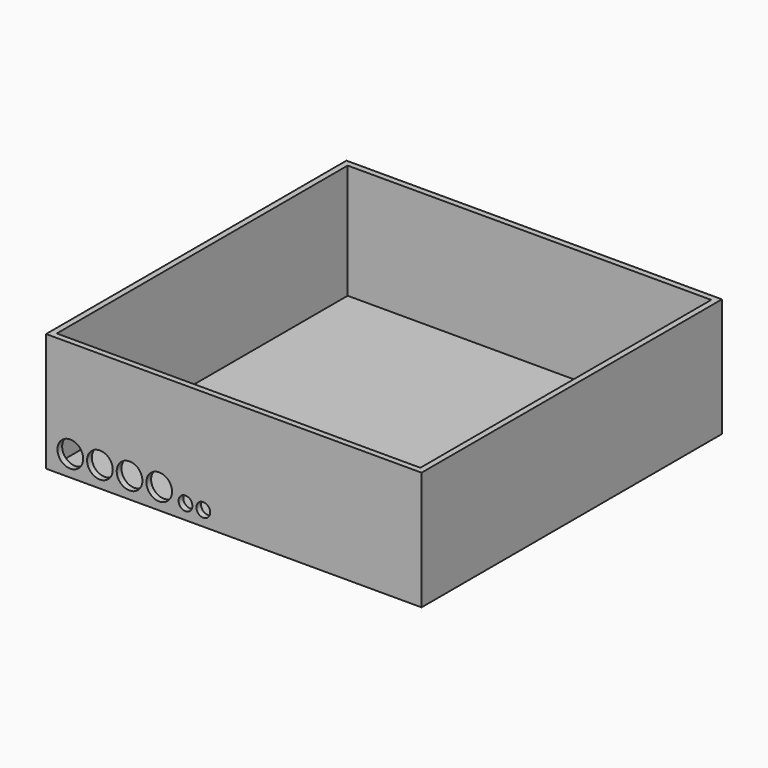
from build123d import *

# Parameters (mm, degrees)
F0_W     = 184
F0_H     = 184
F1_DEPTH = 2
F0_W_2   = 190
F0_H_2   = 190
F2_DEPTH = 60
F3_R     = 3.5
F3_R_2   = 6.5
F4_DEPTH = 4
F5_DEPTH = 3
F6_SIZE  = 2


# Not quite as in the source:
# - a feature names something its author has since deleted; it is built from what else it names


with BuildPart() as f1:
    # F0 (on Top) → F1 (new body)
    with BuildSketch(Plane.XY):
        with Locations((35.6310763971, 41.0211185324)):
            Rectangle(F0_W, F0_H)
    extrude(amount=F1_DEPTH)

    # F0 (on Top) → F2 (join)
    with BuildSketch(Plane.XY):
        with Locations((35.6310763971, 41.0211185324)):
            Rectangle(F0_W_2, F0_H_2)
        with Locations((35.6310763971, 41.0211185324)):
            Rectangle(F0_W, F0_H, mode=Mode.SUBTRACT)
    extrude(amount=F2_DEPTH)

    # F3 (on face) → F4 (cut)
    with BuildSketch(Plane.XZ.offset(53.9788814676)):
        with Locations((20.1768895756, 7.5)):
            Circle(F3_R)
        with Locations((11.1768895756, 7.5)):
            Circle(F3_R)
        with Locations((-32.1242534935, 10.5)):
            Circle(F3_R_2)
        with Locations((-47.1242534935, 10.5)):
            Circle(F3_R_2)
        with Locations((-17.1242534935, 10.5)):
            Circle(F3_R_2)
        with Locations((-2.1242534935, 10.5)):
            Circle(F3_R_2)
    extrude(amount=-F4_DEPTH, mode=Mode.SUBTRACT)

    # F0 (on Top) → F5 (join)
    with BuildSketch(Plane.XY):
        with Locations((35.6310763971, 41.0211185324)):
            Rectangle(F0_W, F0_H)
    extrude(amount=-F5_DEPTH)

    # F6
    f6_edges = [f1.edges().sort_by_distance(p)[0] for p in [
        (127.631076, 41.021119, -3),
        (35.631076, 133.021119, -3),
        (-56.368924, 41.021119, -3),
        (35.631076, -50.978881, -3),
    ]]
    chamfer(f6_edges, length=F6_SIZE)


solid = f1.part
